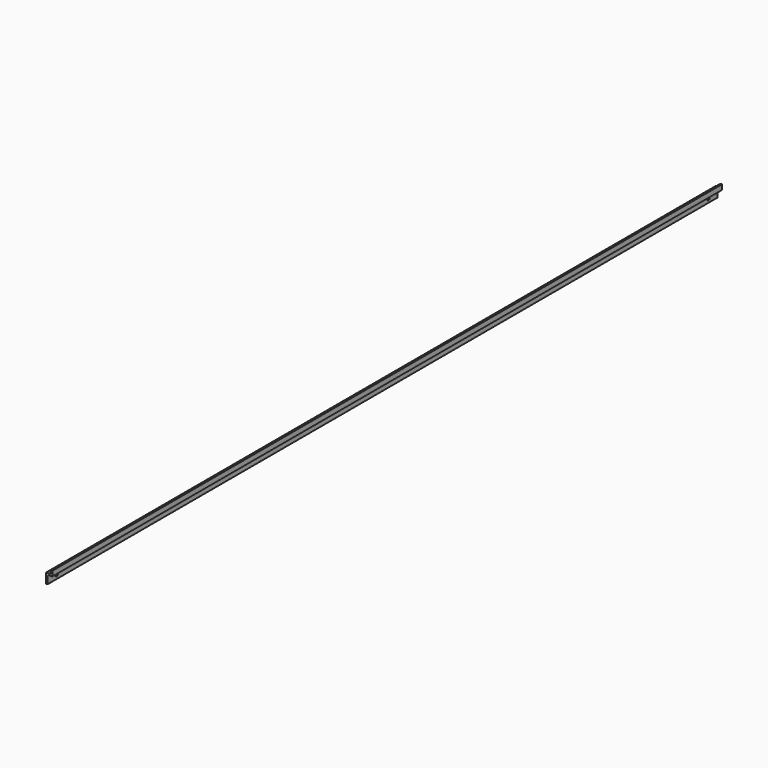
from build123d import *

# Parameters (mm, degrees)
F0_W     = 8.509
F0_H     = 18.3388
F1_DEPTH = 1143
F2_W     = 6.35
F2_H     = 4.7498
F2_H_2   = 11.43
F3_DEPTH = 1143.001
F4_R     = 0.127
F6_DEPTH = 1143.001
F7_R     = 2.032
F8_DEPTH = 2.159


# Not quite as in the source:
# - a pattern or mirror of a feature is missing from the dataset's text; its kind, count and spacing are read off the source's solid


with BuildPart() as f1:
    # F0 (on Front) → F1 (new body)
    with BuildSketch(Plane.XZ):
        with Locations((4.2545, 9.1694)):
            Rectangle(F0_W, F0_H)
    extrude(amount=F1_DEPTH)

    # F2 (on face) → F3 (cut, through all)
    with BuildSketch(Plane.XZ.offset(1143)):
        with Locations((3.175, 15.9639)):
            Rectangle(F2_W, F2_H)
        with Locations((5.334, 5.715)):
            Rectangle(F2_W, F2_H_2)
    extrude(amount=-F3_DEPTH, mode=Mode.SUBTRACT)

    # F4
    f4_edges = [f1.edges().sort_by_distance(p)[0] for p in [
        (6.35, -571.5, 18.3388),
        (8.509, -571.5, 18.3388),
        (2.159, -571.5, 0),
        (0, -571.5, 0),
        (0, -571.5, 13.589),
    ]]
    fillet(f4_edges, radius=F4_R)

    # F7 (on face) → F8 (cut, through all)
    with BuildSketch(Plane.YZ.offset(2.159)):
        with Locations((-1127.76, 5.08)):
            Circle(F7_R)
        with Locations((-15.24, 5.08)):
            Circle(F7_R)
    extrude(amount=-F8_DEPTH, mode=Mode.SUBTRACT)


with BuildPart() as f6:
    # F5 (on face) → F6 (new body, through all)
    with BuildSketch(Plane.XZ.offset(1143)):
        Polygon((2.159, 10.16), (3.683, 11.43), (2.159, 11.43), align=None)
    extrude(amount=-F6_DEPTH)

    # F6_copies: F6 across plane


with BuildPart() as f6_1:
    add(f6.part)
    add(f6.part.mirror(Plane.ZX.offset(-571.405612)))


solid = Compound([f1.part, f6_1.part])
